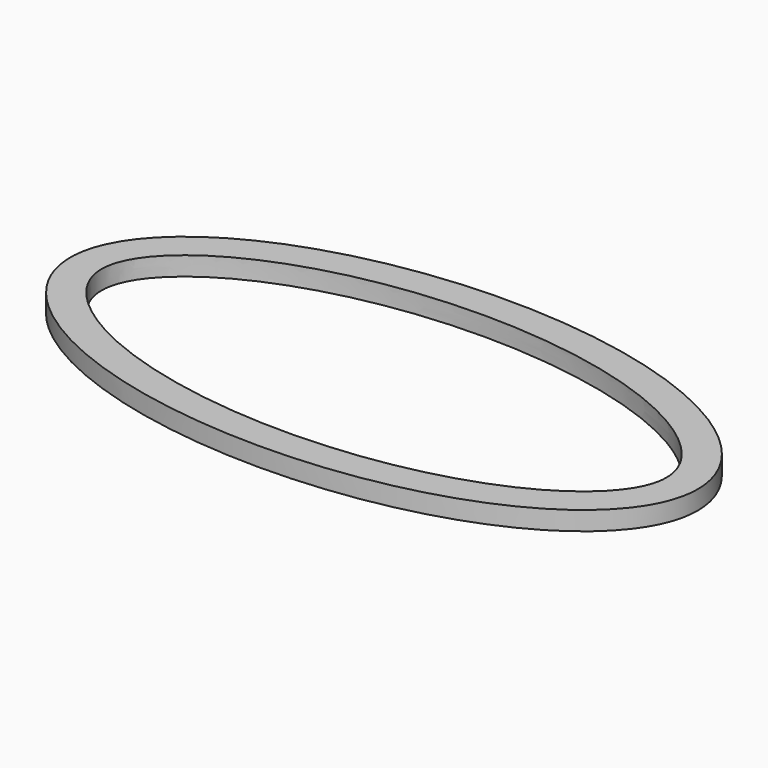
from build123d import *

# Parameters (mm, degrees)
F1_DEPTH = 3


# Not quite as in the source:
# - the dataset's text gives a spline's control points without its knots; the knots are read off the source's solid


with BuildPart() as f1:
    # F0 (on Top) → F1 (new body)
    with BuildSketch(Plane.XY):
        with BuildLine():
            add(Edge.make_bspline(
                [(50, 0), (50, 43.3012701892), (-25, 21.6506350946), (-100, 0), (-25, -21.6506350946), (50, -43.3012701892), (50, 0)],
                knots=[0, 0, 0, 2.0943951024, 2.0943951024, 4.1887902048, 4.1887902048, 6.2831853072, 6.2831853072, 6.2831853072], degree=2, weights=[1, 0.5, 1, 0.5, 1, 0.5, 1]))
        make_face()
        with BuildLine():
            add(Edge.make_bspline(
                [(45.0000010431, 0), (45.0000010431, 0.4960895654), (44.9026405083, 1.4882686963), (44.4473354541, 3.028657329), (43.6338599659, 4.6601234969), (42.4155925881, 6.3701016273), (40.7647525973, 8.1233059984), (38.6726616823, 9.8765449972), (36.5644927344, 11.3035371766), (34.6658260132, 12.4060836573), (33.1350012637, 13.2107562875), (31.5097982219, 13.9840982386), (29.2371951304, 14.9629903055), (26.2034839847, 16.0859961387), (22.2939870458, 17.2556411081), (18.1525453136, 18.2345058178), (13.8165250474, 19.0113864007), (9.3229798868, 19.5766567228), (5.4768533159, 19.8642554217), (2.3586315208, 19.9804484511), (0, 20.0097773391), (-2.3586315208, 19.9804484511), (-5.4768533159, 19.8642554217), (-9.3229798868, 19.5766567228), (-13.8165250474, 19.0113864007), (-18.1525453136, 18.2345058178), (-22.2939870458, 17.2556411081), (-26.2034839847, 16.0859961387), (-29.2371951304, 14.9629903055), (-31.5097982219, 13.9840982386), (-33.1350012637, 13.2107562875), (-34.6658260132, 12.4060836573), (-36.5644927344, 11.3035371766), (-38.6726616823, 9.8765449972), (-40.7647525973, 8.1233059984), (-42.4155925881, 6.3701016273), (-43.6338599659, 4.6601234969), (-44.4473354541, 3.028657329), (-44.9026405083, 1.4882686963), (-45.0486813105, 0), (-44.9026405083, -1.4882686963), (-44.4473354541, -3.028657329), (-43.6338599659, -4.6601234969), (-42.4155925881, -6.3701016273), (-40.7647525973, -8.1233059984), (-38.6726616823, -9.8765449972), (-36.5644927344, -11.3035371766), (-34.6658260132, -12.4060836573), (-33.1350012637, -13.2107562875), (-31.5097982219, -13.9840982386), (-29.2371951304, -14.9629903055), (-26.2034839847, -16.0859961387), (-22.2939870458, -17.2556411081), (-18.1525453136, -18.2345058178), (-13.8165250474, -19.0113864007), (-9.3229798868, -19.5766567228), (-5.4768533159, -19.8642554217), (-2.3586315208, -19.9804484511), (0, -20.0097773391), (2.3586315208, -19.9804484511), (5.4768533159, -19.8642554217), (9.3229798868, -19.5766567228), (13.8165250474, -19.0113864007), (18.1525453136, -18.2345058178), (22.2939870458, -17.2556411081), (26.2034839847, -16.0859961387), (29.2371951304, -14.9629903055), (31.5097982219, -13.9840982386), (33.1350012637, -13.2107562875), (34.6658260132, -12.4060836573), (36.5644927344, -11.3035371766), (38.6726616823, -9.8765449972), (40.7647525973, -8.1233059984), (42.4155925881, -6.3701016273), (43.6338599659, -4.6601234969), (44.4473354541, -3.028657329), (44.9026405083, -1.4882686963), (45.0000010431, -0.4960895654), (45.0000010431, 0)],
                knots=[0, 0, 0, 0, 0.015625, 0.03125, 0.046875, 0.0625, 0.078125, 0.09375, 0.109375, 0.1171875, 0.125, 0.1328125, 0.140625, 0.15625, 0.171875, 0.1875, 0.203125, 0.21875, 0.234375, 0.2421875, 0.25, 0.2578125, 0.265625, 0.28125, 0.296875, 0.3125, 0.328125, 0.34375, 0.359375, 0.3671875, 0.375, 0.3828125, 0.390625, 0.40625, 0.421875, 0.4375, 0.453125, 0.46875, 0.484375, 0.5, 0.515625, 0.53125, 0.546875, 0.5625, 0.578125, 0.59375, 0.609375, 0.6171875, 0.625, 0.6328125, 0.640625, 0.65625, 0.671875, 0.6875, 0.703125, 0.71875, 0.734375, 0.7421875, 0.75, 0.7578125, 0.765625, 0.78125, 0.796875, 0.8125, 0.828125, 0.84375, 0.859375, 0.8671875, 0.875, 0.8828125, 0.890625, 0.90625, 0.921875, 0.9375, 0.953125, 0.96875, 0.984375, 1, 1, 1, 1], degree=3))
        make_face(mode=Mode.SUBTRACT)
    extrude(amount=F1_DEPTH)


solid = f1.part
